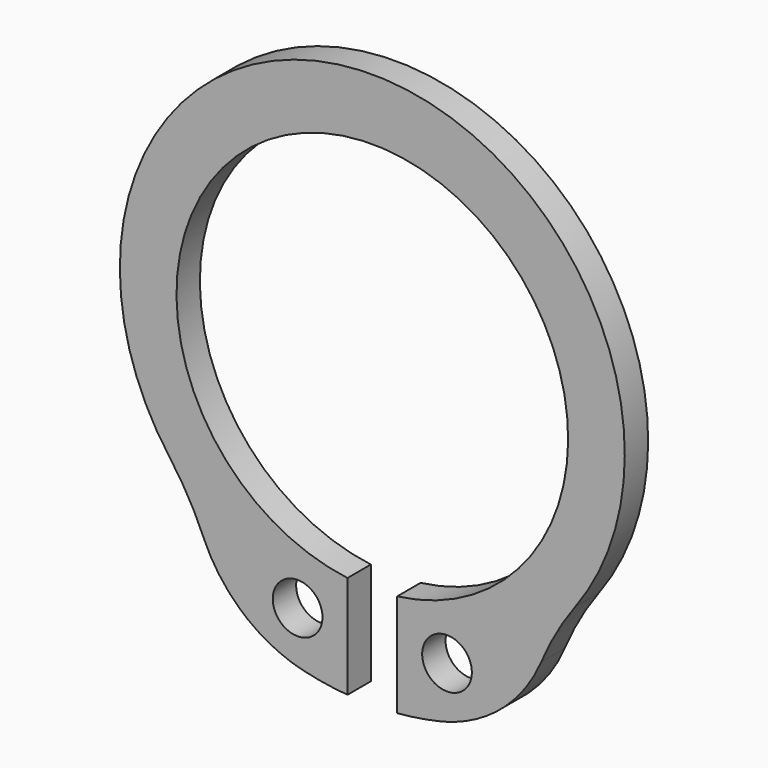
from build123d import *

# Parameters (mm, degrees)
F0_R        = 0.85
F1_DEPTH    = 1
F2_T1_DEPTH = 1
F3_R        = 5


# Not quite as in the source:
# - a fillet or chamfer that OpenCascade refuses, or shapes differently, is made with other operations: its cross-section is extruded or revolved along the edge and cut away or added


with BuildPart() as f1:
    # F0 (on Front) → F1 (new body)
    with BuildSketch(Plane.XZ):
        with BuildLine():
            ThreePointArc((-0.85, -6.6458633751), (0, 6.7), (0.85, -6.6458633751))
            Line((0.85, -6.6458633751), (0.85, -10.1645216316))
            ThreePointArc((0.85, -10.1645216316), (3.1164454592, -9.7122483339), (5.2228952278, -8.7613563698))
            Line((5.2228952278, -8.7613563698), (4.5, -7.2111025509))
            ThreePointArc((4.5, -7.2111025509), (0, 8.8), (-4.5, -7.2111025509))
            Line((-4.5, -7.2111025509), (-5.2228952278, -8.7613563698))
            ThreePointArc((-5.2228952278, -8.7613563698), (-3.1164454592, -9.7122483339), (-0.85, -10.1645216316))
            Line((-0.85, -10.1645216316), (-0.85, -6.6458633751))
        make_face()
        with Locations((-2.5559992958, -8.1065940814)):
            Circle(F0_R, mode=Mode.SUBTRACT)
        with Locations((2.5559992958, -8.1065940814)):
            Circle(F0_R, mode=Mode.SUBTRACT)
    extrude(amount=F1_DEPTH)

    # F2: fillet of radius 10 on 2 edges, made by hand

    # F2_s2 → F2_t1 (join)
    with BuildSketch(Plane.XZ):
        with BuildLine():
            ThreePointArc((-6.9462853719, -4.9724032485), (-5.8852649135, -6.7762174559), (-5.2228952278, -8.7613563698))
            Line((-5.2228952278, -8.7613563698), (-4.5, -7.2111025509))
            ThreePointArc((-4.5, -7.2111025509), (-5.8315783323, -6.210243371), (-6.9462853719, -4.9724032485))
        make_face()
        with BuildLine():
            ThreePointArc((5.2228952278, -8.7613563698), (5.8852649135, -6.7762174559), (6.9462853719, -4.9724032485))
            ThreePointArc((6.9462853719, -4.9724032485), (5.8315783323, -6.210243371), (4.5, -7.2111025509))
            Line((4.5, -7.2111025509), (5.2228952278, -8.7613563698))
        make_face()
    extrude(amount=F2_T1_DEPTH)

    # F3
    f3_edges = [f1.edges().sort_by_distance(p)[0] for p in [
        (-5.222895, -0.5, -8.761356),
        (5.222895, -0.5, -8.761356),
    ]]
    fillet(f3_edges, radius=F3_R)


solid = f1.part
